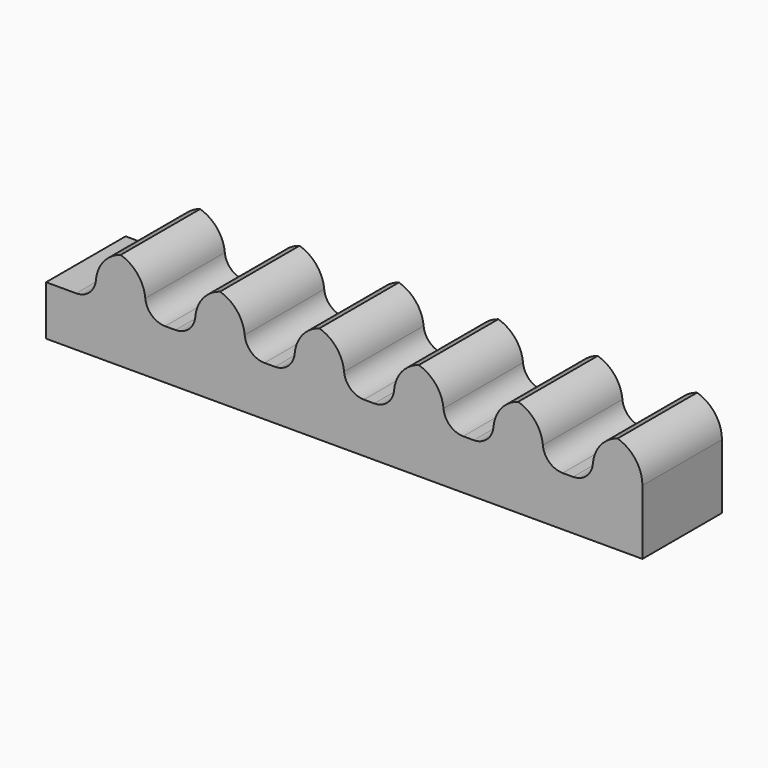
from build123d import *

# Parameters (mm, degrees)
F0_W        = 12.7
F0_H        = 12.7
F1_DEPTH    = 25.4
F2_T1_DEPTH = 69.85
F3_R        = 5.08


# Not quite as in the source:
# - a fillet or chamfer that OpenCascade refuses, or shapes differently, is made with other operations: its cross-section is extruded or revolved along the edge and cut away or added


with BuildPart() as f1:
    # F0 (on Front) → F1 (new body)
    with BuildSketch(Plane.XZ):
        Polygon((12.7, 0), (0, 0), (-12.7, 0), (-25.4, 0), (-38.1, 0), (-50.8, 0), (-63.5, 0), (-76.2, 0), (-76.2, -12.7), (0, -12.7), (76.2, -12.7), (76.2, 0), (63.5, 0), (50.8, 0), (38.1, 0), (25.4, 0), align=None)
        with Locations((-6.35, 6.35)):
            Rectangle(F0_W, F0_H)
        with Locations((19.05, 6.35)):
            Rectangle(F0_W, F0_H)
        with Locations((-31.75, 6.35)):
            Rectangle(F0_W, F0_H)
        with Locations((44.45, 6.35)):
            Rectangle(F0_W, F0_H)
        with Locations((-57.15, 6.35)):
            Rectangle(F0_W, F0_H)
        with Locations((69.85, 6.35)):
            Rectangle(F0_W, F0_H)
    extrude(amount=F1_DEPTH)

    # F2: fillet of radius 8.89 on 12 edges, made by hand

    # F2_s2 → F2_t1 (cut)
    with BuildSketch(Plane.XZ.offset(-22.225)):
        with BuildLine():
            ThreePointArc((-54.61, 12.7), (-60.8961792847, 10.0961792847), (-63.5, 3.81))
            Line((-63.5, 3.81), (-63.5, 12.7))
            Line((-63.5, 12.7), (-54.61, 12.7))
        make_face()
        with BuildLine():
            ThreePointArc((-50.8, 3.81), (-53.4038207153, 10.0961792847), (-59.69, 12.7))
            Line((-59.69, 12.7), (-50.8, 12.7))
            Line((-50.8, 12.7), (-50.8, 3.81))
        make_face()
        with BuildLine():
            ThreePointArc((-29.21, 12.7), (-35.4961792847, 10.0961792847), (-38.1, 3.81))
            Line((-38.1, 3.81), (-38.1, 12.7))
            Line((-38.1, 12.7), (-29.21, 12.7))
        make_face()
        with BuildLine():
            ThreePointArc((-25.4, 3.81), (-28.0038207153, 10.0961792847), (-34.29, 12.7))
            Line((-34.29, 12.7), (-25.4, 12.7))
            Line((-25.4, 12.7), (-25.4, 3.81))
        make_face()
        with BuildLine():
            ThreePointArc((-3.81, 12.7), (-10.0961792847, 10.0961792847), (-12.7, 3.81))
            Line((-12.7, 3.81), (-12.7, 12.7))
            Line((-12.7, 12.7), (-3.81, 12.7))
        make_face()
        with BuildLine():
            ThreePointArc((0, 3.81), (-2.6038207153, 10.0961792847), (-8.89, 12.7))
            Line((-8.89, 12.7), (0, 12.7))
            Line((0, 12.7), (0, 3.81))
        make_face()
        with BuildLine():
            ThreePointArc((21.59, 12.7), (15.3038207153, 10.0961792847), (12.7, 3.81))
            Line((12.7, 3.81), (12.7, 12.7))
            Line((12.7, 12.7), (21.59, 12.7))
        make_face()
        with BuildLine():
            ThreePointArc((25.4, 3.81), (22.7961792847, 10.0961792847), (16.51, 12.7))
            Line((16.51, 12.7), (25.4, 12.7))
            Line((25.4, 12.7), (25.4, 3.81))
        make_face()
        with BuildLine():
            ThreePointArc((46.99, 12.7), (40.7038207153, 10.0961792847), (38.1, 3.81))
            Line((38.1, 3.81), (38.1, 12.7))
            Line((38.1, 12.7), (46.99, 12.7))
        make_face()
        with BuildLine():
            ThreePointArc((50.8, 3.81), (48.1961792847, 10.0961792847), (41.91, 12.7))
            Line((41.91, 12.7), (50.8, 12.7))
            Line((50.8, 12.7), (50.8, 3.81))
        make_face()
        with BuildLine():
            ThreePointArc((76.2, 3.81), (73.5961792847, 10.0961792847), (67.31, 12.7))
            Line((67.31, 12.7), (76.2, 12.7))
            Line((76.2, 12.7), (76.2, 3.81))
        make_face()
        with BuildLine():
            ThreePointArc((72.39, 12.7), (66.1038207153, 10.0961792847), (63.5, 3.81))
            Line((63.5, 3.81), (63.5, 12.7))
            Line((63.5, 12.7), (72.39, 12.7))
        make_face()
    extrude(amount=F2_T1_DEPTH, mode=Mode.SUBTRACT)

    # F3
    f3_edges = [f1.edges().sort_by_distance(p)[0] for p in [
        (-63.5, -12.7, 0),
        (-50.8, -12.7, 0),
        (-38.1, -12.7, 0),
        (-25.4, -12.7, 0),
        (-12.7, -12.7, 0),
        (0, -12.7, 0),
        (12.7, -12.7, 0),
        (38.1, -12.7, 0),
        (63.5, -12.7, 0),
        (50.8, -12.7, 0),
        (25.4, -12.7, 0),
    ]]
    fillet(f3_edges, radius=F3_R)


solid = f1.part
